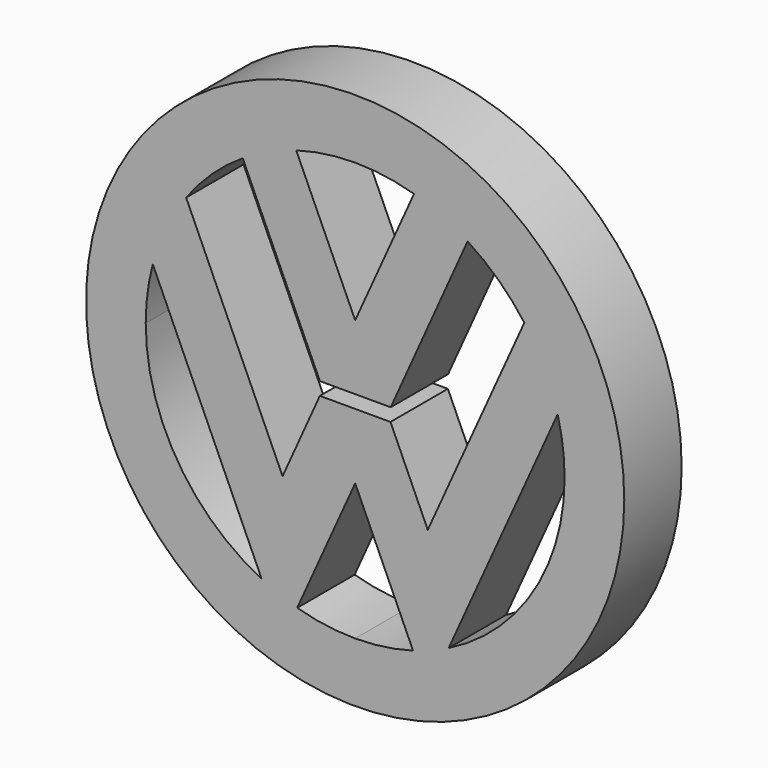
from build123d import *

# Parameters (mm, degrees)
F1_DEPTH = 2


# Not quite as in the source:
# - ends of sketch curves that miss each other by under 0.0002 mm in the source are joined


with BuildPart() as f1:
    # F0 (on Front) → F1 (new body)
    with BuildSketch(Plane.XZ):
        with BuildLine():
            ThreePointArc((-7.5, 0), (0, -7.5), (7.5, 0))
            ThreePointArc((7.5, 0), (0, 7.5), (-7.5, 0))
        make_face()
        with BuildLine():
            ThreePointArc((-9.252e-06, -5.837642026), (-0.8154481123, -5.781304427), (-1.6149720231, -5.6113751006))
            Line((-1.6149720231, -5.6113751006), (0, -2.0297722424))
            Line((0, -2.0297722424), (1.6130763481, -5.6119564271))
            ThreePointArc((1.6130763481, -5.6119564271), (0.8143893667, -5.7809478456), (-9.252e-06, -5.837642026))
        make_face(mode=Mode.SUBTRACT)
        with BuildLine():
            ThreePointArc((-5.8376432623, 4.535e-07), (-5.7885795806, 0.7619262356), (-5.6402209677, 1.5108774116))
            Line((-5.6402209677, 1.5108774116), (-2.6057938378, -5.2253115461))
            ThreePointArc((-2.6057938378, -5.2253115461), (-4.9642649621, -3.0719201723), (-5.8376432623, 4.535e-07))
        make_face(mode=Mode.SUBTRACT)
        with BuildLine():
            ThreePointArc((5.8375074432, 8.164e-07), (4.9638082552, -3.0717207498), (2.6056583249, -5.2253113695))
            Line((2.6056583249, -5.2253113695), (5.6435948014, 1.498042557))
            ThreePointArc((5.6435948014, 1.498042557), (5.7887533107, 0.7552604254), (5.8375074432, 8.164e-07))
        make_face(mode=Mode.SUBTRACT)
        with BuildLine():
            Line((0, 1.9682461262), (-1.6421023797, 5.6034935248))
            ThreePointArc((-1.6421023797, 5.6034935248), (-0.8294183969, 5.7791792496), (-8.9799e-06, 5.8374974962))
            ThreePointArc((-8.9799e-06, 5.8374974962), (0.8283723862, 5.7788128003), (1.6402065238, 5.6039289974))
            Line((1.6402065238, 5.6039289974), (0, 1.9682461262))
        make_face(mode=Mode.SUBTRACT)
        with BuildLine():
            Line((0.990821727, 0.1571487487), (3.1334508081, 4.9261166556))
            ThreePointArc((3.1334508081, 4.9261166556), (3.9933572695, 4.2579147754), (4.7150061526, 3.4423429304))
            Line((4.7150061526, 3.4423429304), (2.0229239131, -2.5149786417))
            Line((2.0229239131, -2.5149786417), (0.9841275984, -0.2051414777))
            Line((0.9841275984, -0.2051414777), (-0.9841094572, -0.2051414777))
            Line((-0.9841094572, -0.2051414777), (-2.0228967012, -2.5149786417))
            Line((-2.0228967012, -2.5149786417), (-4.7110881859, 3.447911577))
            ThreePointArc((-4.7110881859, 3.447911577), (-3.9911114988, 4.2602728506), (-3.1337140349, 4.925981317))
            Line((-3.1337140349, 4.925981317), (-0.9841094572, 0.1571487487))
            Line((-0.9841094572, 0.1571487487), (0.990821727, 0.1571487487))
        make_face(mode=Mode.SUBTRACT)
    extrude(amount=F1_DEPTH)


solid = f1.part
